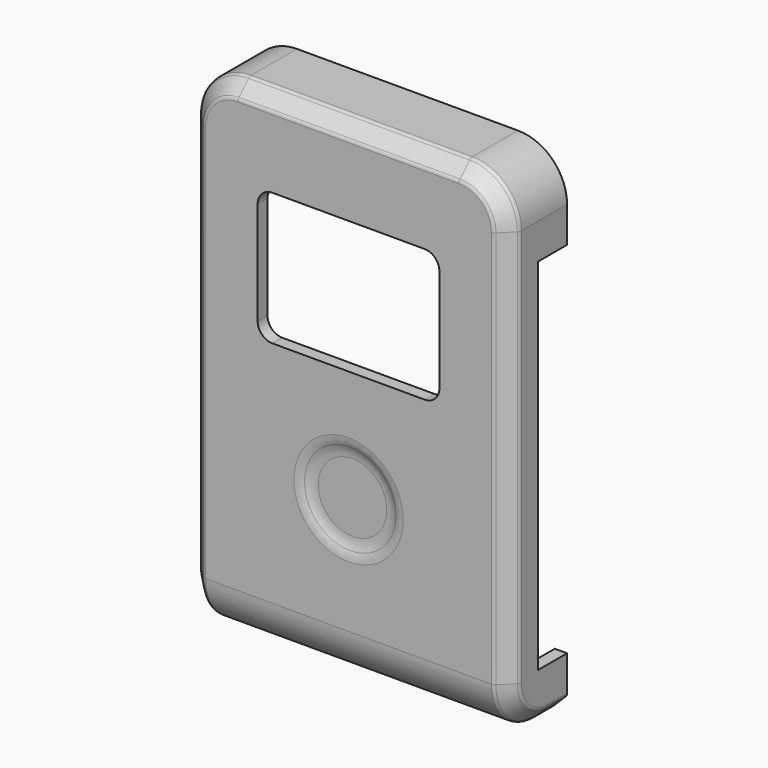
from build123d import *

# Parameters (mm, degrees)
F1_DEPTH  = 15
F2_R      = 10
F3_SIZE   = 3
F4_R      = 1
F6_DEPTH  = 25.4
F7_R      = 10
F8_DEPTH  = 1
F11_T     = -2.5
F12_W     = 7.4454136193
F12_H     = 73.2100643218
F3_FACE_W = 3.4142135624
F3_FACE_H = 81
F13_DEPTH = 81.8


# Not quite as in the source:
# - a fillet or chamfer that OpenCascade refuses, or shapes differently, is made with other operations: its cross-section is extruded or revolved along the edge and cut away or added


with BuildPart() as f1:
    # F0 (on Front) → F1 (new body)
    with BuildSketch(Plane.XZ):
        with BuildLine():
            Line((22.5, 50.5), (-22.5, 50.5))
            ThreePointArc((-22.5, 50.5), (-29.5710678119, 47.5710678119), (-32.5, 40.5))
            Line((-32.5, 40.5), (-32.5, -50.5))
            Line((-32.5, -50.5), (32.5, -50.5))
            Line((32.5, -50.5), (32.5, 40.5))
            ThreePointArc((32.5, 40.5), (29.5710678119, 47.5710678119), (22.5, 50.5))
        make_face()
    extrude(amount=F1_DEPTH)

    # F2
    f2_edges = [f1.edges().sort_by_distance(p)[0] for p in [
        (0, -15, -50.5),
    ]]
    fillet(f2_edges, radius=F2_R)

    # F3
    f3_edges = [f1.edges().sort_by_distance(p)[0] for p in [
        (32.5, -15, 0),
        (-32.5, -2.5, -50.5),
        (-32.5, -12.071068, -47.571068),
        (-32.5, -15, 0),
        (32.5, -2.5, -50.5),
        (32.5, -12.071068, -47.571068),
        (-29.571068, -15, 47.571068),
        (0, -15, 50.5),
        (29.571068, -15, 47.571068),
    ]]
    chamfer(f3_edges, length=F3_SIZE)

    # F4
    f4_edges = [f1.edges().sort_by_distance(p)[0] for p in [
        (32.5, -12, 0),
        (-32.5, -12, 0),
        (29.5, -15, 0),
        (-32.5, -2.5, -47.5),
        (-32.5, -9.949747, -45.449747),
        (-29.5, -2.5, -50.5),
        (-29.571068, -12, 47.571068),
        (-29.5, -12.071068, -47.571068),
        (-29.5, -15, 0),
        (29.5, -2.5, -50.5),
        (0, -12, 50.5),
        (32.5, -2.5, -47.5),
        (29.571068, -12, 47.571068),
        (32.5, -9.949747, -45.449747),
        (-27.449747, -15, 45.449747),
        (29.5, -12.071068, -47.571068),
        (27.449747, -15, 45.449747),
        (0, -15, 47.5),
    ]]
    fillet(f4_edges, radius=F4_R)

    # F5 (on face) → F6 (cut)
    with BuildSketch(Plane.XZ.offset(15)):
        with BuildLine():
            Line((15.5, 33.0857864376), (-15.5, 33.0857864376))
            ThreePointArc((-15.5, 33.0857864376), (-17.6213203436, 32.2071067812), (-18.5, 30.0857864376))
            Line((-18.5, 30.0857864376), (-18.5, 9.0857864376))
            ThreePointArc((-18.5, 9.0857864376), (-17.6213203436, 6.9644660941), (-15.5, 6.0857864376))
            Line((-15.5, 6.0857864376), (15.5, 6.0857864376))
            ThreePointArc((15.5, 6.0857864376), (17.6213203436, 6.9644660941), (18.5, 9.0857864376))
            Line((18.5, 9.0857864376), (18.5, 30.0857864376))
            ThreePointArc((18.5, 30.0857864376), (17.6213203436, 32.2071067812), (15.5, 33.0857864376))
        make_face()
    extrude(amount=-F6_DEPTH, mode=Mode.SUBTRACT)

    # F7 (on face) → F8 (cut)
    with BuildSketch(Plane.XZ.offset(15)):
        with Locations((0, -16.9142135624)):
            Circle(F7_R)
    extrude(amount=-F8_DEPTH, mode=Mode.SUBTRACT)

    # F9: fillet of radius 5.08 on 1 edges, made by hand

    # F9_s1 → F9_t2 (revolve)
    with BuildSketch(Plane.XY.offset(-16.9142135624)):
        with BuildLine():
            ThreePointArc((10, -15), (8.567188555, -14.2564743185), (6.9734508099, -14))
            Line((6.9734508099, -14), (10, -14))
            Line((10, -14), (10, -15))
        make_face()
    revolve(axis=Axis((0, -14, -16.9142135624), (0, -1, 0)))

    # F10: fillet of radius 4 on 1 edges, made by hand

    # F10_s1 → F10_t2 (revolve, cut)
    with BuildSketch(Plane.XY.offset(-16.9142135624)):
        with BuildLine():
            add(Edge.make_bspline(
                [(11.1159138454, -15), (10.1503047462, -15), (9.2910402615, -14.5594713656)],
                knots=[0, 0, 0, 1, 1, 1], degree=2, weights=[1, 1, 1]))
            ThreePointArc((9.2910402615, -14.5594713656), (9.6545831872, -14.7651501561), (10, -15))
            Line((10, -15), (11.1159138454, -15))
        make_face()
    revolve(axis=Axis((0, -15, -16.9142135624), (0, -1, 0)), mode=Mode.SUBTRACT)

    # F11
    f11_openings = [f1.faces().sort_by_distance(p)[0] for p in [
        (18.5, -7.5, 19.585786),
        (17.62132, -7.5, 32.207107),
        (0, -7.5, 33.085786),
        (-17.62132, -7.5, 32.207107),
        (-18.5, -7.5, 19.585786),
        (-17.62132, -7.5, 6.964466),
        (0, -7.5, 6.085786),
        (17.62132, -7.5, 6.964466),
        (0, 0, -3.809825),
    ]]
    offset(amount=F11_T, openings=f11_openings)

    # F12 (on face) + F3_face (on face) → F13 (cut)
    with BuildSketch(Plane(origin=(-32.5, 0, 0), x_dir=(0, -1, 0), z_dir=(-1, 0, 0))):
        with Locations((3.7227068096, -3.3467467874)):
            Rectangle(F12_W, F12_H)
    with BuildSketch(Plane(origin=(31, -13.5, 0), x_dir=(0.7071067812, 0.7071067812, 0), z_dir=(0.7071067812, -0.7071067812, 0))):
        Rectangle(F3_FACE_W, F3_FACE_H)
    extrude(amount=-F13_DEPTH, dir=(-1, 0, 0), mode=Mode.SUBTRACT)


solid = f1.part
